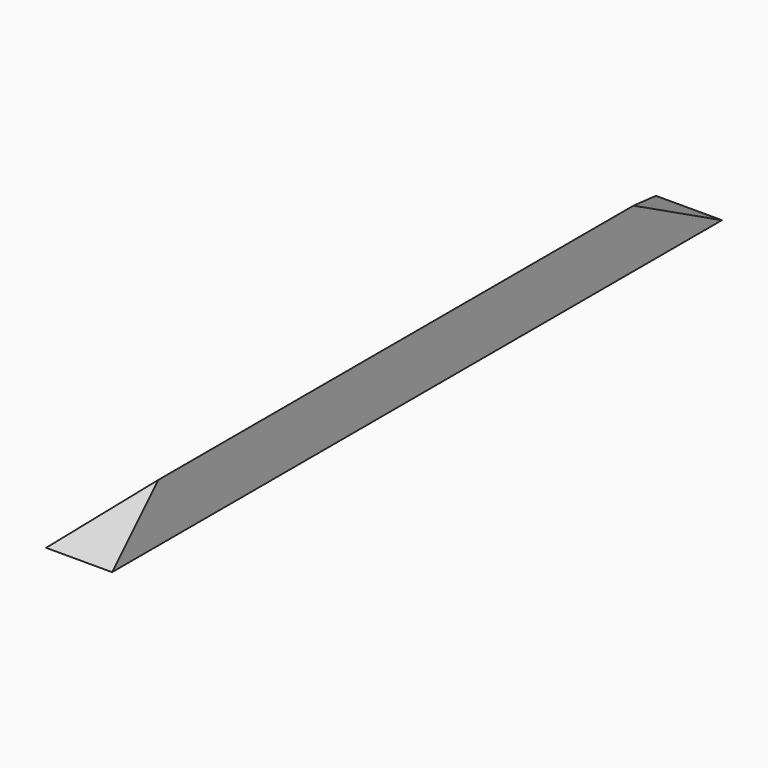
from build123d import *

# Parameters (mm, degrees)
F0_W     = 20
F0_H     = 231
F1_DEPTH = 8.75
F2_SIZE2 = 17.49999
F2_SIZE  = 17.49999
F3_SIZE2 = 33.49999
F3_SIZE  = 17.49999
F4_SIZE2 = 17.49999
F4_SIZE  = 19.99999


# Not quite as in the source:
# - a fillet or chamfer is up to 0.001 mm smaller than in the source, because OpenCascade refuses the exact size


with BuildPart() as f1:
    # F0 (on Top) → F1 (new body, symmetric)
    with BuildSketch(Plane.XY):
        Rectangle(F0_W, F0_H)
    extrude(amount=F1_DEPTH, both=True)

    # F2 (size 17.5 and 17.5 in the source; OpenCascade refuses exactly that, so slightly less here)
    f2_edges = [f1.edges().sort_by_distance(p)[0] for p in [
        (0, -115.5, 8.75),
    ]]
    chamfer(f2_edges, length=F2_SIZE, length2=F2_SIZE2)

    # F3 (size 17.5 and 33.5 in the source; OpenCascade refuses exactly that, so slightly less here)
    f3_edges = [f1.edges().sort_by_distance(p)[0] for p in [
        (0, 115.5, 8.75),
    ]]
    f3_side = f1.faces().sort_by_distance((0, 115.5, 0))[0]
    chamfer(f3_edges, length=F3_SIZE, length2=F3_SIZE2, reference=f3_side)

    # F4 (size 20 and 17.5 in the source; OpenCascade refuses exactly that, so slightly less here)
    f4_edges = [f1.edges().sort_by_distance(p)[0] for p in [
        (-10, -8, 8.75),
    ]]
    f4_side = f1.faces().sort_by_distance((0, -8, 8.75))[0]
    chamfer(f4_edges, length=F4_SIZE, length2=F4_SIZE2, reference=f4_side)


solid = f1.part
